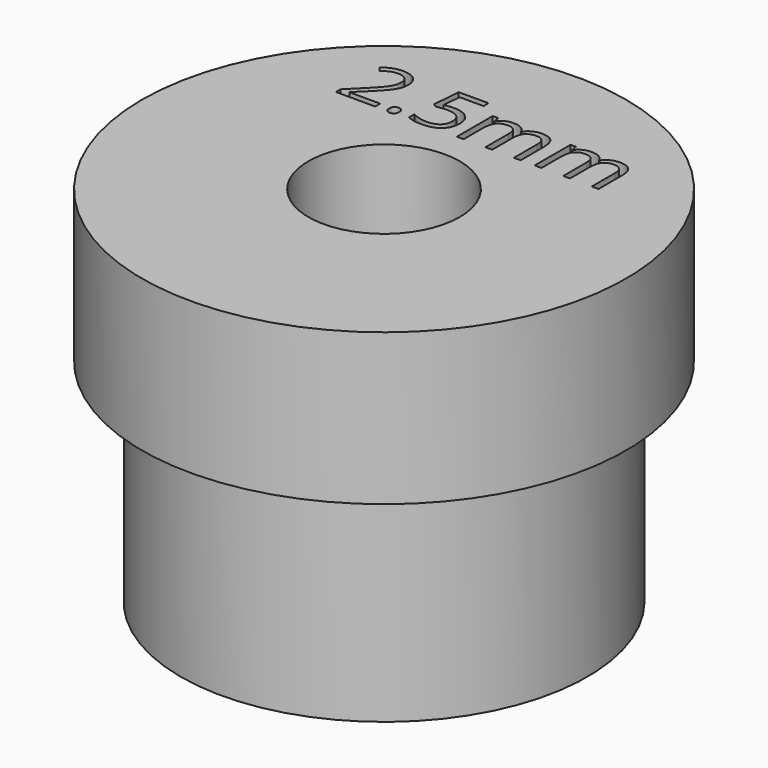
from build123d import *

# Parameters (mm, degrees)
F2_R         = 1.25
F3_DEPTH     = 25
F2_TEXT_SIZE = 1.3820178356
F4_DEPTH     = 1.5


# Not quite as in the source:
# - a feature names something its author has since deleted; it is built from what else it names
# - Text() gives the source's letters only with a copy of the font that has no kerning and outlines rounded to 1/6400 em; it was checked with that copy


with BuildPart() as f1:
    # F0 (on Front) → F1 (revolve)
    with BuildSketch(Plane.XZ):
        Polygon((0, -1.25), (0, 0), (-4, 0), (-4, -2.5), (-3.36, -2.5), (-3.36, -6), align=None)
    revolve(axis=Axis((0, 0, -0.625), (0, 0, 1)))

    # F2 (on face) → F3 (cut)
    with BuildSketch(Plane.XY):
        Circle(F2_R)
    extrude(amount=-F3_DEPTH, mode=Mode.SUBTRACT)

    # F2 (on face) → F4 (cut)
    with BuildSketch(Plane.XY):
        Circle(F2_R)
        with Locations((-2.2482622961, 1.7307870061)):
            Text('2.5mm', F2_TEXT_SIZE, font='Open Sans', text_align=(TextAlign.LEFT, TextAlign.BOTTOM))
    extrude(amount=-F4_DEPTH, mode=Mode.SUBTRACT)


solid = f1.part
